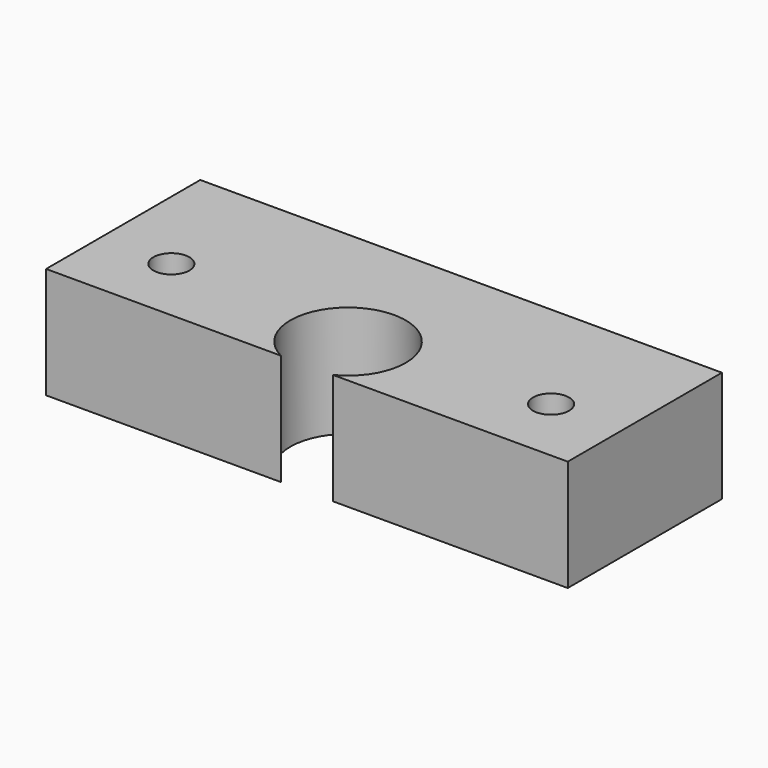
from build123d import *

# Parameters (mm, degrees)
F0_R     = 2.0574
F1_DEPTH = 12.7


# Not quite as in the source:
# - a feature names something its author has since deleted; it is built from what else it names


with BuildPart() as f1:
    # F0 (on Top) → F1 (new body)
    with BuildSketch(Plane.XY):
        with BuildLine():
            Line((0, 8.9704120984), (0, -13.0232248562))
            Line((0, -13.0232248562), (26.7917899333, -13.0232248562))
            ThreePointArc((26.7917899333, -13.0232248562), (29.7688, -0.5781617802), (32.7458100667, -13.0232248562))
            Line((32.7458100667, -13.0232248562), (59.5376, -13.0232248562))
            Line((59.5376, -13.0232248562), (59.5376, 8.9704120984))
            Line((59.5376, 8.9704120984), (0, 8.9704120984))
        make_face()
        with Locations((8.1026, -5.2786845261)):
            Circle(F0_R, mode=Mode.SUBTRACT)
        with Locations((51.435, -5.2786845261)):
            Circle(F0_R, mode=Mode.SUBTRACT)
    extrude(amount=F1_DEPTH)


solid = f1.part
